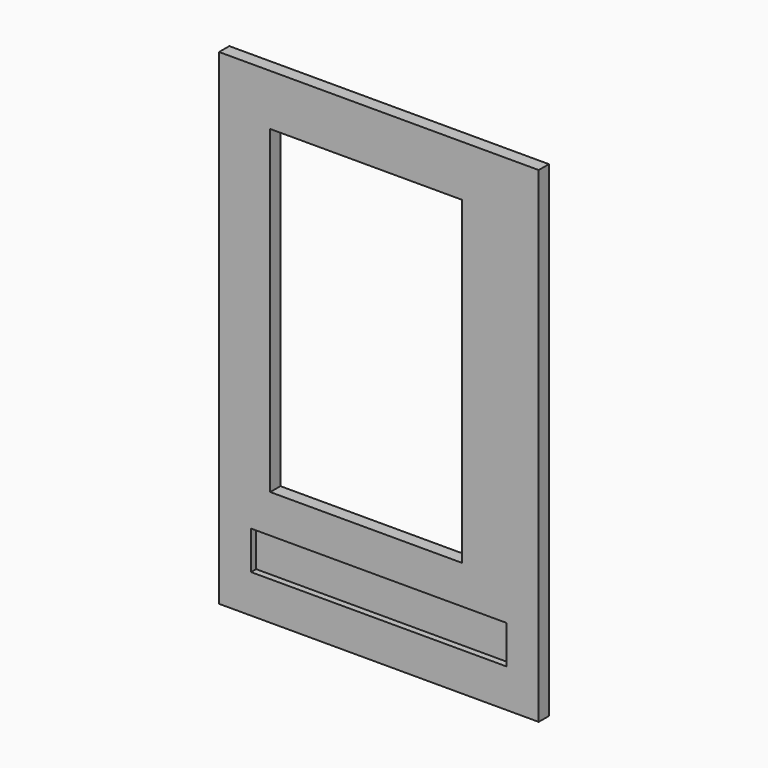
from build123d import *

# Parameters (mm, degrees)
F0_W     = 25
F0_H     = 38
F0_W_2   = 20
F0_H_2   = 3
F0_W_3   = 15
F0_H_3   = 25
F1_DEPTH = 1
F2_W     = 22.4918248132
F2_H     = 4.8074135557
F2_W_2   = 20
F2_H_2   = 3
F3_DEPTH = 0.5


with BuildPart() as f1:
    # F0 (on Front) → F1 (new body)
    with BuildSketch(Plane.XZ):
        Rectangle(F0_W, F0_H)
        with Locations((0, -14.5)):
            Rectangle(F0_W_2, F0_H_2, mode=Mode.SUBTRACT)
        with Locations((-1, 2.5)):
            Rectangle(F0_W_3, F0_H_3, mode=Mode.SUBTRACT)
    extrude(amount=F1_DEPTH)

    # F2 (on face) → F3 (join)
    with BuildSketch(Plane(origin=(0, 0, 0), x_dir=(-1, 0, 0), z_dir=(0, 1, 0))):
        with Locations((0.0546504743, -14.3780573271)):
            Rectangle(F2_W, F2_H)
        with Locations((0, -14.5)):
            Rectangle(F2_W_2, F2_H_2, mode=Mode.SUBTRACT)
        with Locations((0, -14.5)):
            Rectangle(F2_W_2, F2_H_2)
    extrude(amount=-F3_DEPTH)


solid = f1.part
